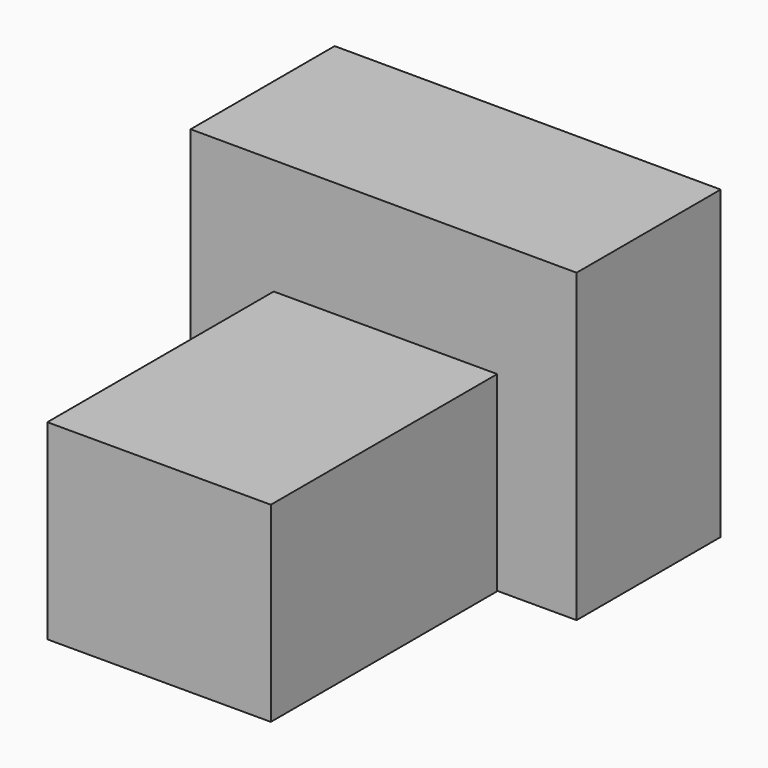
from build123d import *

# Parameters (mm, degrees)
F1_DEPTH = 28.448
F2_W     = 35.3105356917
F2_H     = 30.2078574896
F3_DEPTH = 73.152


# Not quite as in the source:
# - a feature names something its author has since deleted; it is built from what else it names


with BuildPart() as f1:
    # F0 (on Front) → F1 (new body)
    with BuildSketch(Plane.XZ):
        Polygon((21.7242818326, 32.0553742349), (-39.2557755113, 32.1793556213), (-39.2557755113, -16.2723716348), (21.7242818326, -16.2723716348), align=None)
    extrude(amount=F1_DEPTH)

    # F2 (on Front) → F3 (join)
    with BuildSketch(Plane.XZ):
        with Locations((-8.470446337, -1.2246426195)):
            Rectangle(F2_W, F2_H)
    extrude(amount=F3_DEPTH)


solid = f1.part
